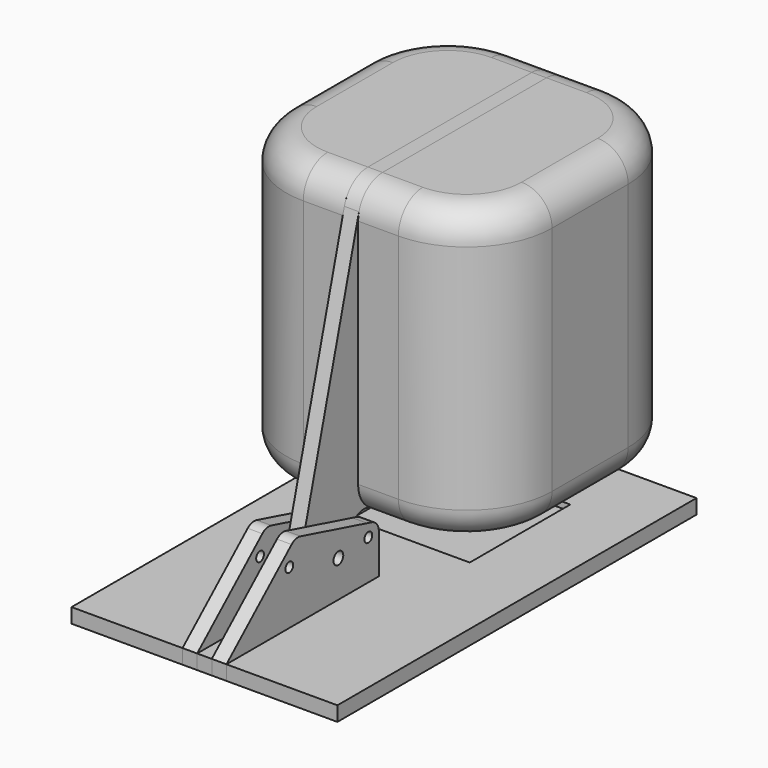
from build123d import *

# Parameters (mm, degrees)
F1_W           = 148
F1_H           = 145
F2_DEPTH       = 103
F3_R           = 70
F4_R           = 25
F6_DEPTH       = 148
F9_R           = 5
F10_DEPTH      = 12
F9_R_2         = 4
F9_W           = 40
F9_H           = 12
F11_DEPTH      = 12
F9_W_2         = 211.7265462875
F9_W_3         = 76.2734537125
F13_DEPTH      = 115
F13_DEPTH_BACK = 103
F14_R          = 10
F14_2_R        = 10
F16_W          = 103
F16_H          = 103
F17_DEPTH      = 5
F18_R          = 15


# Not quite as in the source:
# - a feature names something its author has since deleted; it is built from what else it names


with BuildPart() as f2:
    # F1 (on Right) → F2 (new body)
    with BuildSketch(Plane.YZ):
        Polygon((-35, 0), (0, 0), (0, 240), (-218, 240), (-218, 0), (-183, 0), (-183, 145), (-35, 145), align=None)
        with Locations((-109, 72.5)):
            Rectangle(F1_W, F1_H)
    extrude(amount=F2_DEPTH)

    # F3
    f3_edges = [f2.edges().sort_by_distance(p)[0] for p in [
        (103, 0, 120),
        (103, -218, 120),
    ]]
    fillet(f3_edges, radius=F3_R)

    # F4
    f4_edges = [f2.edges().sort_by_distance(p)[0] for p in [
        (16.5, 0, 240),
        (16.5, 0, 0),
        (16.5, -218, 0),
        (16.5, -218, 240),
    ]]
    fillet(f4_edges, radius=F4_R)

    # F5 (on face) → F6 (cut)
    with BuildSketch(Plane(origin=(0, 0, 0), x_dir=(1, 0, 0), z_dir=(0, 0, -1))):
        with BuildLine():
            Line((0, 193), (0, 25))
            Line((0, 25), (33, 25))
            ThreePointArc((33, 25), (64.8198051534, 38.1801948466), (78, 70))
            Line((78, 70), (78, 148))
            ThreePointArc((78, 148), (64.8198051534, 179.8198051534), (33, 193))
            Line((33, 193), (0, 193))
        make_face()
    extrude(amount=-F6_DEPTH, mode=Mode.SUBTRACT)


with BuildPart() as f2_1:
    # F7: moved
    add(f2.part.moved(Location((6, 0, 0))))


with BuildPart() as f8_1:
    # F8: instance of F2
    add(f2_1.part.mirror(Plane.YZ))


with BuildPart() as f10:
    # F9 (on face) → F10 (new body)
    with BuildSketch(Plane(origin=(6, 0, 0), x_dir=(0, -1, 0), z_dir=(-1, 0, 0))):
        with BuildLine():
            Line((193, 240), (25, 240))
            ThreePointArc((25, 240), (7.3223304703, 232.6776695297), (0, 215))
            Line((0, 215), (0, 25))
            ThreePointArc((0, 25), (7.3223304703, 7.3223304703), (25, 0))
            Line((25, 0), (25, 148))
            Line((25, 148), (193, 148))
            Line((193, 148), (193, 0))
            ThreePointArc((193, 0), (210.6776695297, 7.3223304703), (218, 25))
            Line((218, 25), (218, 215))
            ThreePointArc((218, 215), (217.7863573886, 218.2613628143), (217.1490810075, 221.4669843431))
            ThreePointArc((217.1490810075, 221.4669843431), (208.2204696285, 234.8327331523), (193, 240))
        make_face()
        with BuildLine():
            Line((272.1252428955, 16.1744219246), (217.1490810075, 221.4669843431))
            ThreePointArc((217.1490810075, 221.4669843431), (217.7863573886, 218.2613628143), (218, 215))
            Line((218, 215), (218, 25))
            Line((218, 25), (223.8270808805, 3.2404532384))
            Line((223.8270808805, 3.2404532384), (272.1252428955, 16.1744219246))
        make_face()
        with BuildLine():
            Line((277.4027807961, -3.5330156569), (272.1252428955, 16.1744219246))
            Line((272.1252428955, 16.1744219246), (223.8270808805, 3.2404532384))
            Line((223.8270808805, 3.2404532384), (226.4138746589, -6.4191793184))
            Line((226.4138746589, -6.4191793184), (229.1046187811, -16.4669843431))
            ThreePointArc((229.1046187811, -16.4669843431), (259.7206841317, -34.1490810075), (277.4027807961, -3.5330156569))
        make_face()
        with Locations((253.2536997886, -10)):
            Circle(F9_R, mode=Mode.SUBTRACT)
    extrude(amount=F10_DEPTH)

    # F18
    f18_edges = [f10.edges().sort_by_distance(p)[0] for p in [
        (0, -218, 25),
    ]]
    fillet(f18_edges, radius=F18_R)


with BuildPart() as f11:
    # F9 (on face) → F11 (new body)
    with BuildSketch(Plane(origin=(6, 0, 0), x_dir=(0, -1, 0), z_dir=(-1, 0, 0))):
        with BuildLine():
            Line((277.4027807961, -3.5330156569), (272.1252428955, 16.1744219246))
            Line((272.1252428955, 16.1744219246), (223.8270808805, 3.2404532384))
            Line((223.8270808805, 3.2404532384), (226.4138746589, -6.4191793184))
            Line((226.4138746589, -6.4191793184), (229.1046187811, -16.4669843431))
            ThreePointArc((229.1046187811, -16.4669843431), (259.7206841317, -34.1490810075), (277.4027807961, -3.5330156569))
        make_face()
        with Locations((253.2536997886, -10)):
            Circle(F9_R, mode=Mode.SUBTRACT)
        with BuildLine():
            Line((297.1817845062, 22.8844189733), (272.1252428955, 16.1744219246))
            Line((272.1252428955, 16.1744219246), (277.4027807961, -3.5330156569))
            ThreePointArc((277.4027807961, -3.5330156569), (259.7206841317, -34.1490810075), (229.1046187811, -16.4669843431))
            Line((229.1046187811, -16.4669843431), (226.4138746589, -6.4191793184))
            Line((226.4138746589, -6.4191793184), (223.8270808805, 3.2404532384))
            Line((223.8270808805, 3.2404532384), (211.7265462875, 0))
            Line((211.7265462875, 0), (211.7265462875, -40))
            Line((211.7265462875, -40), (251.7265462875, -40))
            Line((251.7265462875, -40), (328, -40))
            Line((328, -40), (368, -40))
            Line((368, -40), (297.1817845062, 22.8844189733))
        make_face()
        with BuildLine():
            ThreePointArc((226.5500216565, -7.4538966595), (218.584204464, -7.9757146308), (226.4138746589, -6.4191793184))
            ThreePointArc((226.4138746589, -6.4191793184), (226.5158388491, -6.9320786881), (226.5500216565, -7.4538966595))
        make_face(mode=Mode.SUBTRACT)
        with Locations((303.5250168082, 3.8783782931)):
            Circle(F9_R_2, mode=Mode.SUBTRACT)
        with Locations((348, -46)):
            Rectangle(F9_W, F9_H)
        with Locations((231.7265462875, -46)):
            Rectangle(F9_W, F9_H)
    extrude(amount=-F11_DEPTH)


with BuildPart() as f12_1:
    # F12: copy of F11
    add(f11.part.moved(Location((-24, 0, 0))))

    # F14#2
    f14_2_edges = [f12_1.edges().sort_by_distance(p)[0] for p in [
        (-12, -297.181785, 22.884419),
        (-12, -211.726546, 0),
    ]]
    fillet(f14_2_edges, radius=F14_2_R)


with BuildPart() as f13:
    # F9 (on face) → F13 (new body, two sides)
    with BuildSketch(Plane(origin=(6, 0, 0), x_dir=(0, -1, 0), z_dir=(-1, 0, 0))) as f13_sk:
        with Locations((105.8632731438, -46)):
            Rectangle(F9_W_2, F9_H)
        with Locations((231.7265462875, -46)):
            Rectangle(F9_W, F9_H)
        with Locations((289.8632731438, -46)):
            Rectangle(F9_W_3, F9_H)
        with Locations((348, -46)):
            Rectangle(F9_W, F9_H)
    extrude(amount=F13_DEPTH)
    extrude(f13_sk.sketch, amount=-F13_DEPTH_BACK)


with BuildPart() as f11_1:
    add(f11.part)

    # F14
    f14_edges = [f11_1.edges().sort_by_distance(p)[0] for p in [
        (12, -297.181785, 22.884419),
        (12, -211.726546, 0),
    ]]
    fillet(f14_edges, radius=F14_R)


with BuildPart() as f13_1:
    add(f13.part)

    # F15: cut F12_1, F11
    add(f12_1.part, mode=Mode.SUBTRACT)
    add(f11_1.part, mode=Mode.SUBTRACT)

    # F16 (on face) → F17 (cut)
    with BuildSketch(Plane.XY.offset(-40)):
        with Locations((0, -109)):
            Rectangle(F16_W, F16_H)
    extrude(amount=-F17_DEPTH, mode=Mode.SUBTRACT)


solid = Compound([f2_1.part, f8_1.part, f10.part, f12_1.part, f11_1.part, f13_1.part])
